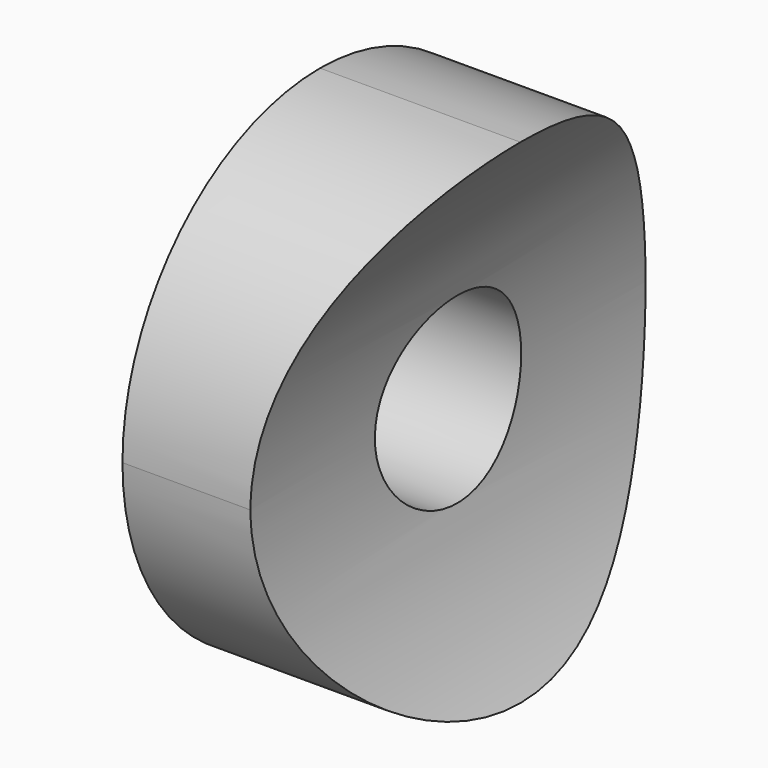
from build123d import *

# Parameters (mm, degrees)
F1_DEPTH = 13.716
F2_R     = 6.8579
F3_R     = 2.54
F4_DEPTH = 5.5678543904


# Not quite as in the source:
# - a fillet or chamfer is up to 0.001 mm smaller than in the source, because OpenCascade refuses the exact size


with BuildPart() as f1:
    # F0 (on Front) → F1 (new body)
    with BuildSketch(Plane.XZ):
        with BuildLine():
            ThreePointArc((-10.6891457096, -6.858), (-12.7, 0), (-10.6891457096, 6.858))
            Line((-10.6891457096, 6.858), (-16.256, 6.858))
            Line((-16.256, 6.858), (-16.256, 0))
            Line((-16.256, 0), (-16.256, -6.858))
            Line((-16.256, -6.858), (-10.6891457096, -6.858))
        make_face()
    extrude(amount=F1_DEPTH)

    # F2 (radius 6.858 in the source; OpenCascade refuses exactly that, so slightly less here)
    f2_edges = [f1.edges().sort_by_distance(p)[0] for p in [
        (-13.472573, 0, 6.858),
        (-13.472573, -13.716, 6.858),
        (-13.472573, -13.716, -6.858),
        (-13.472573, 0, -6.858),
    ]]
    fillet(f2_edges, radius=F2_R)

    # F3 (on face) → F4 (cut, through all)
    with BuildSketch(Plane(origin=(-16.256, 0, 0), x_dir=(0, -1, 0), z_dir=(-1, 0, 0))):
        with Locations((6.858, 0)):
            Circle(F3_R)
    extrude(amount=-F4_DEPTH, mode=Mode.SUBTRACT)


solid = f1.part
